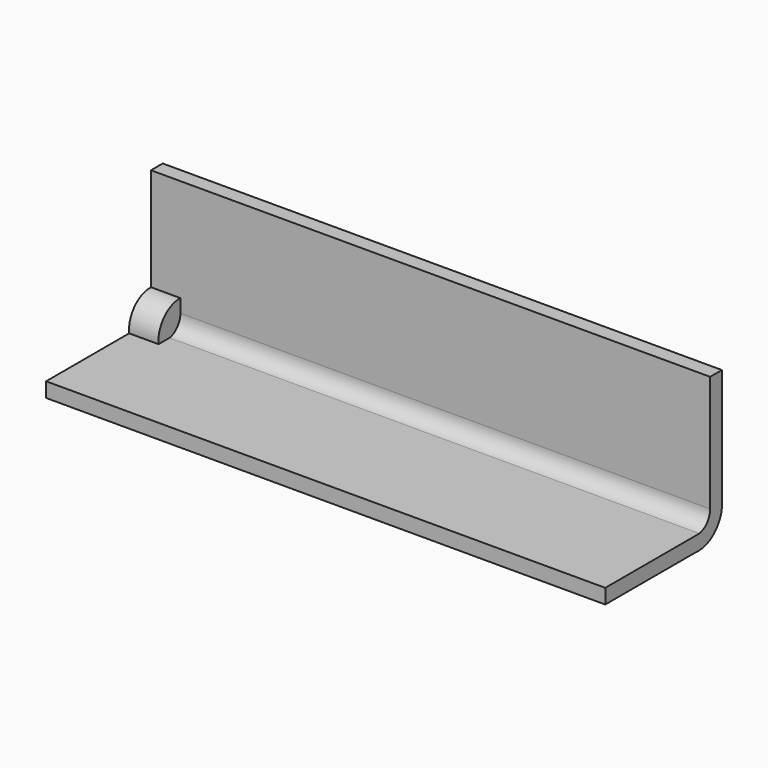
from build123d import *

# Parameters (mm, degrees)
F1_DEPTH = 482.6
F2_R     = 22.9562722026
F3_DEPTH = 25.4


# Not quite as in the source:
# - a feature names something its author has since deleted; it is built from what else it names


with BuildPart() as f1:
    # F0 (on Right) → F1 (new body)
    with BuildSketch(Plane.YZ):
        with BuildLine():
            Line((-812.6182556152, 512.6869344869), (-812.6182556152, 611.3093582153))
            Line((-812.6182556152, 611.3093582153), (-825.3182556152, 611.3093582153))
            Line((-825.3182556152, 611.3093582153), (-825.3182556152, 510.914683342))
            ThreePointArc((-825.3182556152, 510.914683342), (-828.5785642638, 501.8659167533), (-836.8610188459, 496.9760562897))
            Line((-836.8610188459, 496.9760562897), (-938.4610188459, 496.9760562897))
            Line((-938.4610188459, 496.9760562897), (-938.4610188459, 484.2760562897))
            Line((-938.4610188459, 484.2760562897), (-840.6965225196, 484.2760562897))
            ThreePointArc((-840.6965225196, 484.2760562897), (-822.0453350188, 489.7370832304), (-812.6182556152, 506.7317819438))
            ThreePointArc((-812.6182556152, 506.7317819438), (-812.7921868823, 509.7093582153), (-812.6182556152, 512.6869344869))
        make_face()
    extrude(amount=F1_DEPTH)

    # F2 (on Right) → F3 (join)
    with BuildSketch(Plane.YZ):
        with Locations((-826.0604739189, 499.5044767857)):
            Circle(F2_R)
    extrude(amount=F3_DEPTH)


solid = f1.part
